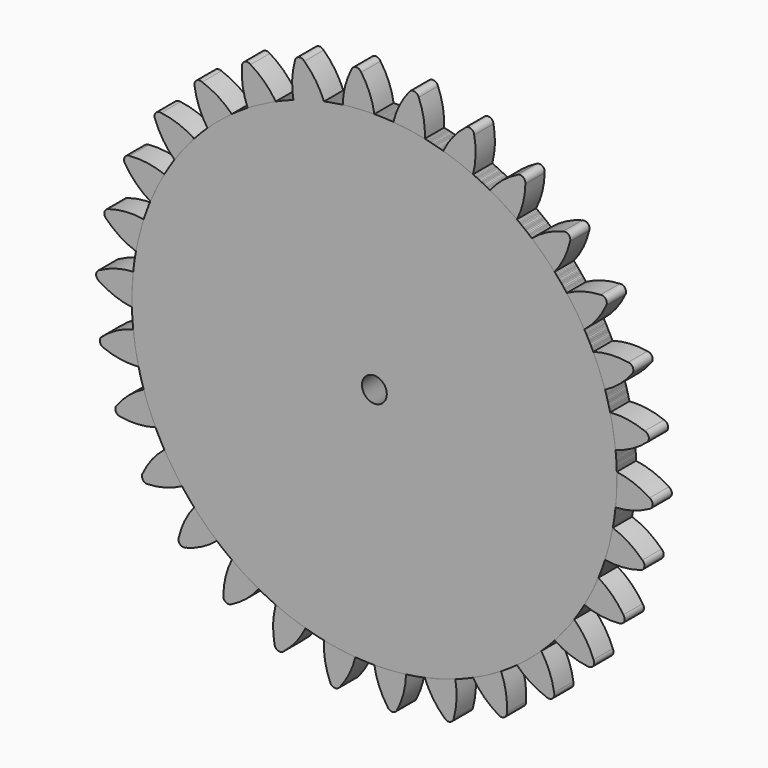
from build123d import *

# Parameters (mm, degrees)
F0_R     = 0.9168797315
F1_DEPTH = 1.778
F2_COUNT = 30


with BuildPart() as f1:
    # F0 (on Front) → F1 (new body)
    with BuildSketch(Plane.XZ):
        with BuildLine():
            ThreePointArc((-2.3365682183, 17.7479976538), (-11.8030446628, -13.4587929789), (17.901144426, 0))
            ThreePointArc((17.901144426, 0), (12.6580206146, 12.6580206146), (0, 17.901144426))
            ThreePointArc((0, 17.901144426), (-1.1707908623, 17.8628167016), (-2.3365682183, 17.7479976538))
        make_face()
        Circle(F0_R, mode=Mode.SUBTRACT)
        with BuildLine():
            ThreePointArc((-2.3365682183, 17.7479976538), (-1.1707908623, 17.8628167016), (0, 17.901144426))
            ThreePointArc((0, 17.901144426), (-0.3474744343, 19.1540298754), (-0.9672816385, 20.2969644586))
            ThreePointArc((-0.9672816385, 20.2969644586), (-1.3444095567, 20.5117260975), (-1.6902790744, 20.249576703))
            ThreePointArc((-1.6902790744, 20.249576703), (-2.155600843, 19.0355190093), (-2.3365682183, 17.7479976538))
        make_face()
    extrude(amount=F1_DEPTH)


with BuildPart() as f2_1:
    # F2: instance of F1
    add(f1.part.rotate(Axis((0, 0, 0), (0, 1, 0)), 1 * 360 / F2_COUNT))


with BuildPart() as f2_2:
    # F2: instance of F1
    add(f1.part.rotate(Axis((0, 0, 0), (0, 1, 0)), 2 * 360 / F2_COUNT))


with BuildPart() as f2_3:
    # F2: instance of F1
    add(f1.part.rotate(Axis((0, 0, 0), (0, 1, 0)), 3 * 360 / F2_COUNT))


with BuildPart() as f2_4:
    # F2: instance of F1
    add(f1.part.rotate(Axis((0, 0, 0), (0, 1, 0)), 4 * 360 / F2_COUNT))


with BuildPart() as f2_5:
    # F2: instance of F1
    add(f1.part.rotate(Axis((0, 0, 0), (0, 1, 0)), 5 * 360 / F2_COUNT))


with BuildPart() as f2_6:
    # F2: instance of F1
    add(f1.part.rotate(Axis((0, 0, 0), (0, 1, 0)), 6 * 360 / F2_COUNT))


with BuildPart() as f2_7:
    # F2: instance of F1
    add(f1.part.rotate(Axis((0, 0, 0), (0, 1, 0)), 7 * 360 / F2_COUNT))


with BuildPart() as f2_8:
    # F2: instance of F1
    add(f1.part.rotate(Axis((0, 0, 0), (0, 1, 0)), 8 * 360 / F2_COUNT))


with BuildPart() as f2_9:
    # F2: instance of F1
    add(f1.part.rotate(Axis((0, 0, 0), (0, 1, 0)), 9 * 360 / F2_COUNT))


with BuildPart() as f2_10:
    # F2: instance of F1
    add(f1.part.rotate(Axis((0, 0, 0), (0, 1, 0)), 10 * 360 / F2_COUNT))


with BuildPart() as f2_11:
    # F2: instance of F1
    add(f1.part.rotate(Axis((0, 0, 0), (0, 1, 0)), 11 * 360 / F2_COUNT))


with BuildPart() as f2_12:
    # F2: instance of F1
    add(f1.part.rotate(Axis((0, 0, 0), (0, 1, 0)), 12 * 360 / F2_COUNT))


with BuildPart() as f2_13:
    # F2: instance of F1
    add(f1.part.rotate(Axis((0, 0, 0), (0, 1, 0)), 13 * 360 / F2_COUNT))


with BuildPart() as f2_14:
    # F2: instance of F1
    add(f1.part.rotate(Axis((0, 0, 0), (0, 1, 0)), 14 * 360 / F2_COUNT))


with BuildPart() as f2_15:
    # F2: instance of F1
    add(f1.part.rotate(Axis((0, 0, 0), (0, 1, 0)), 15 * 360 / F2_COUNT))


with BuildPart() as f2_16:
    # F2: instance of F1
    add(f1.part.rotate(Axis((0, 0, 0), (0, 1, 0)), 16 * 360 / F2_COUNT))


with BuildPart() as f2_17:
    # F2: instance of F1
    add(f1.part.rotate(Axis((0, 0, 0), (0, 1, 0)), 17 * 360 / F2_COUNT))


with BuildPart() as f2_18:
    # F2: instance of F1
    add(f1.part.rotate(Axis((0, 0, 0), (0, 1, 0)), 18 * 360 / F2_COUNT))


with BuildPart() as f2_19:
    # F2: instance of F1
    add(f1.part.rotate(Axis((0, 0, 0), (0, 1, 0)), 19 * 360 / F2_COUNT))


with BuildPart() as f2_20:
    # F2: instance of F1
    add(f1.part.rotate(Axis((0, 0, 0), (0, 1, 0)), 20 * 360 / F2_COUNT))


with BuildPart() as f2_21:
    # F2: instance of F1
    add(f1.part.rotate(Axis((0, 0, 0), (0, 1, 0)), 21 * 360 / F2_COUNT))


with BuildPart() as f2_22:
    # F2: instance of F1
    add(f1.part.rotate(Axis((0, 0, 0), (0, 1, 0)), 22 * 360 / F2_COUNT))


with BuildPart() as f2_23:
    # F2: instance of F1
    add(f1.part.rotate(Axis((0, 0, 0), (0, 1, 0)), 23 * 360 / F2_COUNT))


with BuildPart() as f2_24:
    # F2: instance of F1
    add(f1.part.rotate(Axis((0, 0, 0), (0, 1, 0)), 24 * 360 / F2_COUNT))


with BuildPart() as f2_25:
    # F2: instance of F1
    add(f1.part.rotate(Axis((0, 0, 0), (0, 1, 0)), 25 * 360 / F2_COUNT))


with BuildPart() as f2_26:
    # F2: instance of F1
    add(f1.part.rotate(Axis((0, 0, 0), (0, 1, 0)), 26 * 360 / F2_COUNT))


with BuildPart() as f2_27:
    # F2: instance of F1
    add(f1.part.rotate(Axis((0, 0, 0), (0, 1, 0)), 27 * 360 / F2_COUNT))


with BuildPart() as f2_28:
    # F2: instance of F1
    add(f1.part.rotate(Axis((0, 0, 0), (0, 1, 0)), 28 * 360 / F2_COUNT))


with BuildPart() as f2_29:
    # F2: instance of F1
    add(f1.part.rotate(Axis((0, 0, 0), (0, 1, 0)), 29 * 360 / F2_COUNT))


solid = Compound([f1.part, f2_1.part, f2_2.part, f2_3.part, f2_4.part, f2_5.part, f2_6.part, f2_7.part, f2_8.part, f2_9.part, f2_10.part, f2_11.part, f2_12.part, f2_13.part, f2_14.part, f2_15.part, f2_16.part, f2_17.part, f2_18.part, f2_19.part, f2_20.part, f2_21.part, f2_22.part, f2_23.part, f2_24.part, f2_25.part, f2_26.part, f2_27.part, f2_28.part, f2_29.part])
